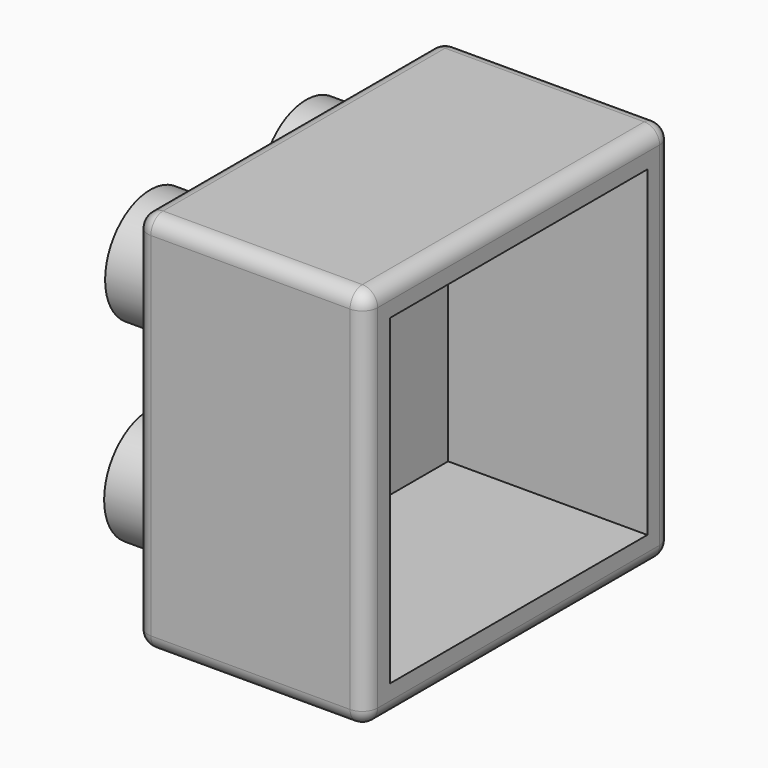
from build123d import *

# Parameters (mm, degrees)
F0_W     = 19.05
F0_H     = 31.75
F1_DEPTH = 31.75
F2_T     = -2.54
F4_R     = 4.6736
F4_R_2   = 3.5941
F5_DEPTH = 5.08
F6_R     = 1.27


# Not quite as in the source:
# - a feature names something its author has since deleted; it is built from what else it names


with BuildPart() as f1:
    # F0 (on Top) → F1 (new body)
    with BuildSketch(Plane.XY):
        with Locations((-14.8217186228, -11.3360365331)):
            Rectangle(F0_W, F0_H)
    extrude(amount=F1_DEPTH)

    # F2
    f2_openings = [f1.faces().sort_by_distance(p)[0] for p in [
        (-5.296719, -11.336037, 15.875),
    ]]
    offset(amount=F2_T, openings=f2_openings)

    # F4 (on face) → F5 (join)
    with BuildSketch(Plane(origin=(-24.3467186228, 0, 0), x_dir=(0, -1, 0), z_dir=(-1, 0, 0))):
        with Locations((19.3370365331, 23.876)):
            Circle(F4_R)
        with Locations((19.3370365331, 23.876)):
            Circle(F4_R_2, mode=Mode.SUBTRACT)
        with Locations((3.2080365331, 23.876)):
            Circle(F4_R)
        with Locations((3.2080365331, 23.876)):
            Circle(F4_R_2, mode=Mode.SUBTRACT)
        with Locations((3.3106288512, 7.8743288743)):
            Circle(F4_R)
        with Locations((3.3106288512, 7.8743288743)):
            Circle(F4_R_2, mode=Mode.SUBTRACT)
        with Locations((19.4396288512, 7.8743288743)):
            Circle(F4_R)
        with Locations((19.4396288512, 7.8743288743)):
            Circle(F4_R_2, mode=Mode.SUBTRACT)
    extrude(amount=F5_DEPTH)

    # F6
    f6_edges = [f1.edges().sort_by_distance(p)[0] for p in [
        (-14.821719, 4.538963, 0),
        (-24.346719, -11.336037, 0),
        (-14.821719, -27.211037, 0),
        (-5.296719, -11.336037, 0),
        (-24.346719, -27.211037, 15.875),
        (-14.821719, 4.538963, 31.75),
        (-24.346719, -11.336037, 31.75),
        (-14.821719, -27.211037, 31.75),
        (-5.296719, -11.336037, 31.75),
        (-5.296719, -27.211037, 15.875),
        (-5.296719, 4.538963, 15.875),
        (-24.346719, 4.538963, 15.875),
    ]]
    fillet(f6_edges, radius=F6_R)


solid = f1.part
